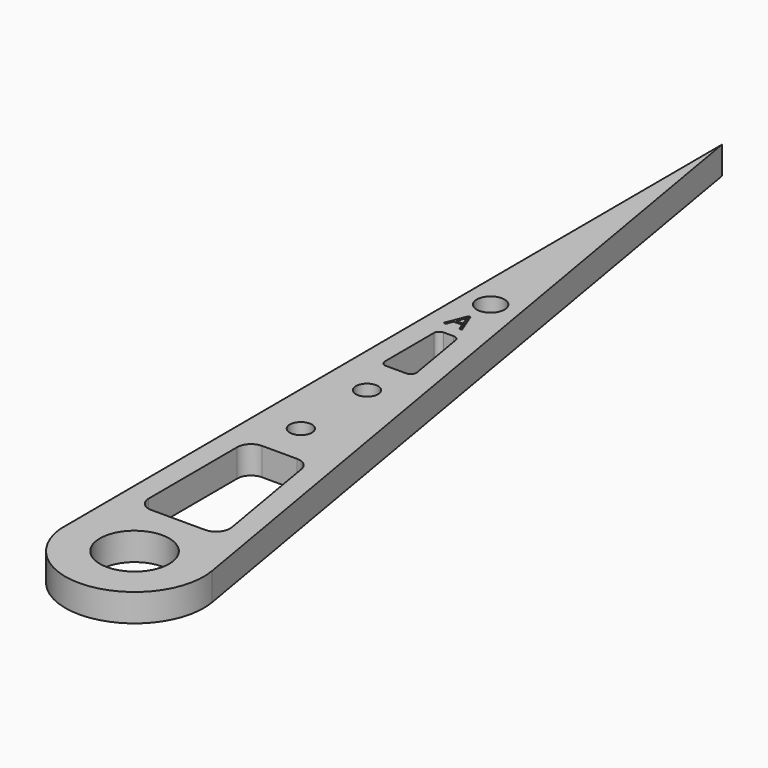
from build123d import *

# Parameters (mm, degrees)
F0_R         = 4
F0_R_2       = 12.5
F0_R_3       = 5
F1_DEPTH     = 10
F2_TEXT_SIZE = 10.6250142886
F3_DEPTH     = 1


# Not quite as in the source:
# - Text() gives the source's letters only with a copy of the font that has no kerning and outlines rounded to 1/6400 em; it was checked with that copy


with BuildPart() as f1:
    # F0 (on Top) → F1 (new body)
    with BuildSketch(Plane.XY):
        with BuildLine():
            Line((-20.5439617748, 242.3022581332), (-19.6348767774, -57.6963644711))
            ThreePointArc((-19.6348767774, -57.6963644711), (8.5964302946, -79.9526971629), (29.8533620733, -50.9614244202))
            Line((29.8533620733, -50.9614244202), (-20.5439617748, 242.3022581332))
        make_face()
        with BuildLine():
            Line((12.6515402426, -32.6197817922), (-6.7259580754, -32.6197817922))
            ThreePointArc((-6.7259580754, -32.6197817922), (-10.2561310823, -31.1606684808), (-11.7259351188, -27.6349332088))
            Line((-11.7259351188, -27.6349332088), (-11.8475099827, 12.4848485834))
            ThreePointArc((-11.8475099827, 12.4848485834), (-10.3884196279, 16.0301730069), (-6.8475329393, 17.5))
            Line((-6.8475329393, 17.5), (5.7569612136, 17.5))
            ThreePointArc((5.7569612136, 17.5), (8.9792136224, 16.3232302329), (10.6847263446, 13.3468357657))
            Line((10.6847263446, 13.3468357657), (17.5793053736, -26.7729460265))
            ThreePointArc((17.5793053736, -26.7729460265), (16.4747704755, -30.8420342009), (12.6515402426, -32.6197817922))
        make_face(mode=Mode.SUBTRACT)
        with Locations((-4.9083716253, 32.5798350328)):
            Circle(F0_R, mode=Mode.SUBTRACT)
        with Locations((-4.9992805424, 62.5798350328)):
            Circle(F0_R, mode=Mode.SUBTRACT)
        with Locations((5.2269052738, -55.1934776624)):
            Circle(F0_R_2, mode=Mode.SUBTRACT)
        with Locations((-10.4418803539, 125.2240272848)):
            Circle(F0_R_3, mode=Mode.SUBTRACT)
        with BuildLine():
            Line((-2.713003403, 77.5), (-10.0505766283, 77.5))
            ThreePointArc((-10.0505766283, 77.5), (-11.462645831, 78.0836453246), (-12.0505674456, 79.4939394334))
            Line((-12.0505674456, 79.4939394334), (-12.1176135283, 101.6191890192))
            ThreePointArc((-12.1176135283, 101.6191890192), (-11.5339773864, 103.0373187886), (-10.117622711, 103.6252495858))
            Line((-10.117622711, 103.6252495858), (-6.5152245267, 103.6252495858))
            ThreePointArc((-6.5152245267, 103.6252495858), (-5.2263235632, 103.154541679), (-4.5441184743, 101.9639838921))
            Line((-4.5441184743, 101.9639838921), (-0.7418973507, 79.8387343063))
            ThreePointArc((-0.7418973507, 79.8387343063), (-1.1837113099, 78.2110990365), (-2.713003403, 77.5))
        make_face(mode=Mode.SUBTRACT)
    extrude(amount=F1_DEPTH)

    # F2 (on face) → F3 (cut)
    with BuildSketch(Plane.XY.offset(10)):
        with Locations((-13.8690238819, 108.116351068)):
            Text('A', F2_TEXT_SIZE, font='Open Sans', text_align=(TextAlign.LEFT, TextAlign.BOTTOM))
    extrude(amount=-F3_DEPTH, mode=Mode.SUBTRACT)


solid = f1.part
